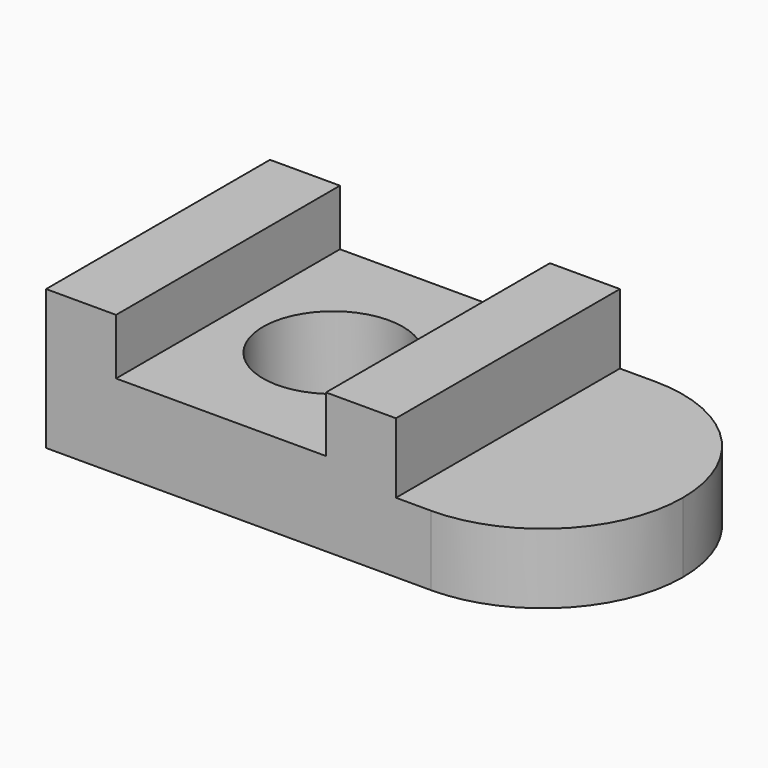
from build123d import *

# Parameters (mm, degrees)
F1_DEPTH = 40
F2_R     = 19.99999
F3_R     = 10
F4_DEPTH = 12.001


# Not quite as in the source:
# - a fillet or chamfer is up to 0.001 mm smaller than in the source, because OpenCascade refuses the exact size


with BuildPart() as f1:
    # F0 (on Front) → F1 (new body)
    with BuildSketch(Plane.XZ):
        Polygon((0, 20), (0, 0), (75, 0), (75, 10), (50, 10), (50, 20), (40, 20), (40, 12), (10, 12), (10, 20), align=None)
    extrude(amount=F1_DEPTH)

    # F2 (radius 20 in the source; OpenCascade refuses exactly that, so slightly less here)
    f2_edges = [f1.edges().sort_by_distance(p)[0] for p in [
        (75, -40, 5),
        (75, 0, 5),
    ]]
    fillet(f2_edges, radius=F2_R)

    # F3 (on face) → F4 (cut, through all)
    with BuildSketch(Plane.XY.offset(12)):
        with Locations((25, -20)):
            Circle(F3_R)
    extrude(amount=-F4_DEPTH, mode=Mode.SUBTRACT)


solid = f1.part
